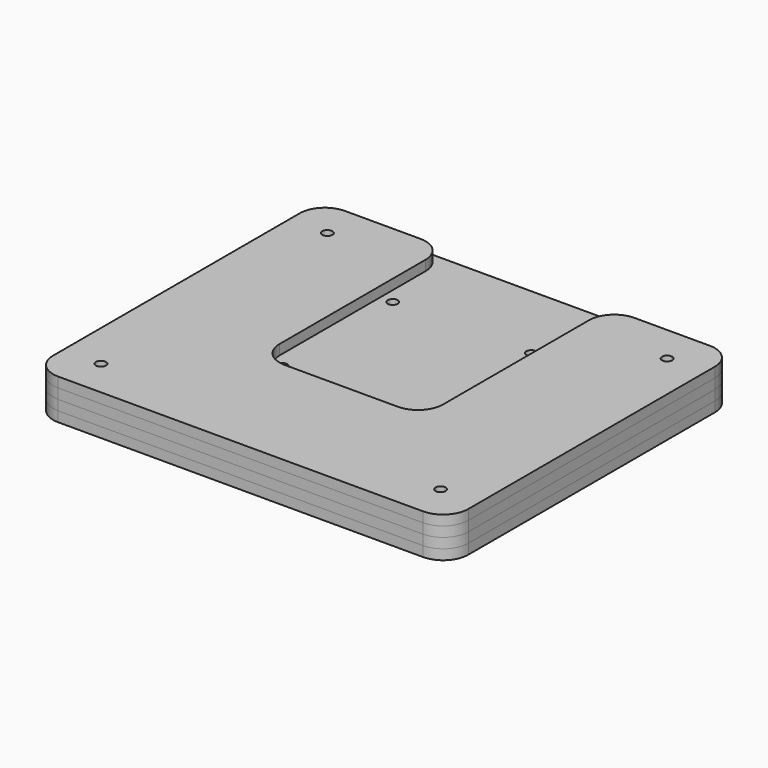
from build123d import *

# Parameters (mm, degrees)
F0_W          = 120
F0_H          = 120
F0_R          = 2
F1_DEPTH      = 4
F2_R          = 10
F3_R          = 4
F4_DEPTH      = 4
F5_W          = 75
F5_H          = 75
F6_DEPTH      = 4
F7_R          = 10
F9_DEPTH      = 4
F10_R         = 4
F10_R_2       = 2
F11_DEPTH     = 4
F12_DEPTH     = 16.001
F13_R         = 2
F14_DEPTH     = 4
F16_DEPTH     = 4
F17_R         = 10
F19_DEPTH     = 4
F20_R         = 10
F22_DEPTH     = 4
F24_DEPTH     = 4
F25_R         = 2
F26_DEPTH     = 16.001
F27_R         = 5
F28_DEPTH     = 8
F30_R         = 2
F31_DEPTH     = 4
F32_TEXT_SIZE = 22.9472929365
F33_DEPTH     = 1
F34_TEXT_SIZE = 22.9472929365
F35_DEPTH     = 1
F36_TEXT_SIZE = 22.9472929365
F37_DEPTH     = 1
F38_TEXT_SIZE = 22.9472929365
F39_DEPTH     = 1
F40_TEXT_SIZE = 22.9472929365
F41_DEPTH     = 1
F42_TEXT_SIZE = 22.9472929365
F43_DEPTH     = 1
F44_TEXT_SIZE = 20.3196105408
F45_DEPTH     = 1
F46_TEXT_SIZE = 20.3196105408
F47_DEPTH     = 1
F48_TEXT_SIZE = 20.3196105408
F49_DEPTH     = 1
F50_TEXT_SIZE = 20.3196105408
F51_DEPTH     = 1


# Not quite as in the source:
# - Text() gives the source's letters only with a copy of the font that has no kerning and outlines rounded to 1/6400 em; it was checked with that copy


with BuildPart() as f1:
    # F0 (on Top) → F1 (new body)
    with BuildSketch(Plane.XY):
        Rectangle(F0_W, F0_H)
        with Locations((-50, -50)):
            Circle(F0_R, mode=Mode.SUBTRACT)
        with Locations((50, -50)):
            Circle(F0_R, mode=Mode.SUBTRACT)
        with Locations((-50, 50)):
            Circle(F0_R, mode=Mode.SUBTRACT)
        with Locations((50, 50)):
            Circle(F0_R, mode=Mode.SUBTRACT)
    extrude(amount=F1_DEPTH)

    # F2
    f2_edges = [f1.edges().sort_by_distance(p)[0] for p in [
        (-60, 60, 2),
        (60, 60, 2),
        (-60, -60, 2),
        (60, -60, 2),
    ]]
    fillet(f2_edges, radius=F2_R)

    # F10 (on face) → F11 (cut, through all)
    with BuildSketch(Plane(origin=(0, 0, 0), x_dir=(1, 0, 0), z_dir=(0, 0, -1))):
        with Locations((27.5, -27.5)):
            Circle(F10_R)
        with Locations((27.5, -27.5)):
            Circle(F10_R_2, mode=Mode.SUBTRACT)
        with Locations((-27.5, -27.5)):
            Circle(F10_R)
        with Locations((-27.5, -27.5)):
            Circle(F10_R_2, mode=Mode.SUBTRACT)
        with Locations((-27.5, 27.5)):
            Circle(F10_R)
        with Locations((-27.5, 27.5)):
            Circle(F10_R_2, mode=Mode.SUBTRACT)
        with Locations((27.5, 27.5)):
            Circle(F10_R)
        with Locations((27.5, 27.5)):
            Circle(F10_R_2, mode=Mode.SUBTRACT)
        with Locations((27.5, -27.5)):
            Circle(F10_R_2)
        with Locations((-27.5, -27.5)):
            Circle(F10_R_2)
        with Locations((-27.5, 27.5)):
            Circle(F10_R_2)
        with Locations((27.5, 27.5)):
            Circle(F10_R_2)
    extrude(amount=-F11_DEPTH, mode=Mode.SUBTRACT)


with BuildPart() as f4:
    # F3 (on face) → F4 (new body)
    with BuildSketch(Plane.XY.offset(4)):
        with BuildLine():
            ThreePointArc((-60, -50), (-57.0710678119, -57.0710678119), (-50, -60))
            Line((-50, -60), (50, -60))
            ThreePointArc((50, -60), (57.0710678119, -57.0710678119), (60, -50))
            Line((60, -50), (60, 50))
            ThreePointArc((60, 50), (57.0710678119, 57.0710678119), (50, 60))
            Line((50, 60), (-50, 60))
            ThreePointArc((-50, 60), (-57.0710678119, 57.0710678119), (-60, 50))
            Line((-60, 50), (-60, -50))
        make_face()
        with Locations((-50, -50)):
            Circle(F3_R, mode=Mode.SUBTRACT)
        with Locations((50, -50)):
            Circle(F3_R, mode=Mode.SUBTRACT)
        with Locations((-50, 50)):
            Circle(F3_R, mode=Mode.SUBTRACT)
        with Locations((50, 50)):
            Circle(F3_R, mode=Mode.SUBTRACT)
    extrude(amount=F4_DEPTH)


with BuildPart() as f6:
    # F5 (on face) → F6 (new body)
    with BuildSketch(Plane.XY.offset(8)):
        Rectangle(F5_W, F5_H)
    extrude(amount=F6_DEPTH)

    # F7
    f7_edges = [f6.edges().sort_by_distance(p)[0] for p in [
        (-37.5, 37.5, 10),
        (37.5, 37.5, 10),
        (37.5, -37.5, 10),
        (-37.5, -37.5, 10),
    ]]
    fillet(f7_edges, radius=F7_R)


with BuildPart() as f9:
    # F8 (on face) → F9 (new body)
    with BuildSketch(Plane.XY.offset(12)):
        with BuildLine():
            ThreePointArc((-60, -50), (-57.0710678119, -57.0710678119), (-50, -60))
            Line((-50, -60), (50, -60))
            ThreePointArc((50, -60), (57.0710678119, -57.0710678119), (60, -50))
            Line((60, -50), (60, 50))
            ThreePointArc((60, 50), (57.0710678119, 57.0710678119), (50, 60))
            Line((50, 60), (-50, 60))
            ThreePointArc((-50, 60), (-57.0710678119, 57.0710678119), (-60, 50))
            Line((-60, 50), (-60, -50))
        make_face()
    extrude(amount=F9_DEPTH)


with BuildPart() as f12_tool:
    # F10 (on face) → F12 (new body, through all)
    with BuildSketch(Plane(origin=(0, 0, 0), x_dir=(1, 0, 0), z_dir=(0, 0, -1))):
        with Locations((27.5, -27.5)):
            Circle(F10_R_2)
        with Locations((-27.5, -27.5)):
            Circle(F10_R_2)
        with Locations((-27.5, 27.5)):
            Circle(F10_R_2)
        with Locations((27.5, 27.5)):
            Circle(F10_R_2)
    extrude(amount=-F12_DEPTH)


with BuildPart() as f4_1:
    add(f4.part)

    # F12: cut by f12_tool
    add(f12_tool.part, mode=Mode.SUBTRACT)

    # F36 (on face) → F37 (cut)
    with BuildSketch(Plane(origin=(0, 0, 4), x_dir=(1, 0, 0), z_dir=(0, 0, -1))):
        with Locations((-15, -8.2610254572)):
            Text('3-1', F36_TEXT_SIZE, font='Open Sans', text_align=(TextAlign.LEFT, TextAlign.BOTTOM))
    extrude(amount=-F37_DEPTH, mode=Mode.SUBTRACT)


with BuildPart() as f6_1:
    add(f6.part)

    # F12: cut by f12_tool
    add(f12_tool.part, mode=Mode.SUBTRACT)

    # F38 (on face) → F39 (cut)
    with BuildSketch(Plane(origin=(0, 0, 8), x_dir=(1, 0, 0), z_dir=(0, 0, -1))):
        with Locations((-15, -8.2610254572)):
            Text('4-1', F38_TEXT_SIZE, font='Open Sans', text_align=(TextAlign.LEFT, TextAlign.BOTTOM))
    extrude(amount=-F39_DEPTH, mode=Mode.SUBTRACT)


with BuildPart() as f9_1:
    add(f9.part)

    # F12: cut by f12_tool
    add(f12_tool.part, mode=Mode.SUBTRACT)


with BuildPart() as f14:
    # F13 (on face) → F14 (new body)
    with BuildSketch(Plane.XY.offset(16)):
        with BuildLine():
            ThreePointArc((-50, 60), (-57.0710678119, 57.0710678119), (-60, 50))
            Line((-60, 50), (-60, -50))
            ThreePointArc((-60, -50), (-57.0710678119, -57.0710678119), (-50, -60))
            Line((-50, -60), (50, -60))
            ThreePointArc((50, -60), (57.0710678119, -57.0710678119), (60, -50))
            Line((60, -50), (60, 50))
            ThreePointArc((60, 50), (57.0710678119, 57.0710678119), (50, 60))
            Line((50, 60), (-50, 60))
        make_face()
        with Locations((-27.5, -27.5)):
            Circle(F13_R, mode=Mode.SUBTRACT)
        with Locations((27.5, -27.5)):
            Circle(F13_R, mode=Mode.SUBTRACT)
        with Locations((-27.5, 27.5)):
            Circle(F13_R, mode=Mode.SUBTRACT)
        with Locations((27.5, 27.5)):
            Circle(F13_R, mode=Mode.SUBTRACT)
    extrude(amount=F14_DEPTH)


with BuildPart() as f16:
    # F15 (on face) → F16 (new body)
    with BuildSketch(Plane.XY.offset(20)):
        Polygon((32.5, -32.5), (0, -32.5), (-32.5, -32.5), (-32.5, 60), (-82.5, 60), (-82.5, -82.5), (0, -82.5), (82.5, -82.5), (82.5, 60), (32.5, 60), align=None)
    extrude(amount=F16_DEPTH)

    # F17
    f17_edges = [f16.edges().sort_by_distance(p)[0] for p in [
        (-32.5, 60, 22),
        (82.5, 60, 22),
        (82.5, -82.5, 22),
        (-32.5, -32.5, 22),
        (-82.5, 60, 22),
        (32.5, 60, 22),
        (32.5, -32.5, 22),
        (-82.5, -82.5, 22),
    ]]
    fillet(f17_edges, radius=F17_R)


with BuildPart() as f19:
    # F18 (on face) → F19 (new body)
    with BuildSketch(Plane(origin=(0, 0, 20), x_dir=(1, 0, 0), z_dir=(0, 0, -1))):
        with BuildLine():
            ThreePointArc((50, 60), (57.0710678119, 57.0710678119), (60, 50))
            Line((60, 50), (60, -50))
            Line((60, -50), (60, -60))
            Line((60, -60), (72.5, -60))
            ThreePointArc((72.5, -60), (79.5710678119, -57.0710678119), (82.5, -50))
            Line((82.5, -50), (82.5, 72.5))
            ThreePointArc((82.5, 72.5), (79.5710678119, 79.5710678119), (72.5, 82.5))
            Line((72.5, 82.5), (-72.5, 82.5))
            ThreePointArc((-72.5, 82.5), (-79.5710678119, 79.5710678119), (-82.5, 72.5))
            Line((-82.5, 72.5), (-82.5, -50))
            ThreePointArc((-82.5, -50), (-79.5710678119, -57.0710678119), (-72.5, -60))
            Line((-72.5, -60), (-60, -60))
            Line((-60, -60), (-60, -50))
            Line((-60, -50), (-60, 50))
            ThreePointArc((-60, 50), (-57.0710678119, 57.0710678119), (-50, 60))
            Line((-50, 60), (50, 60))
        make_face()
    extrude(amount=F19_DEPTH)

    # F20
    f20_edges = [f19.edges().sort_by_distance(p)[0] for p in [
        (-60, 60, 18),
        (60, 60, 18),
    ]]
    fillet(f20_edges, radius=F20_R)


with BuildPart() as f22:
    # F21 (on face) → F22 (new body)
    with BuildSketch(Plane(origin=(0, 0, 16), x_dir=(1, 0, 0), z_dir=(0, 0, -1))):
        with BuildLine():
            ThreePointArc((50, 60), (57.0710678119, 57.0710678119), (60, 50))
            Line((60, 50), (60, -50))
            ThreePointArc((60, -50), (62.9289321881, -57.0710678119), (70, -60))
            Line((70, -60), (72.5, -60))
            ThreePointArc((72.5, -60), (79.5710678119, -57.0710678119), (82.5, -50))
            Line((82.5, -50), (82.5, 72.5))
            ThreePointArc((82.5, 72.5), (79.5710678119, 79.5710678119), (72.5, 82.5))
            Line((72.5, 82.5), (-72.5, 82.5))
            ThreePointArc((-72.5, 82.5), (-79.5710678119, 79.5710678119), (-82.5, 72.5))
            Line((-82.5, 72.5), (-82.5, -50))
            ThreePointArc((-82.5, -50), (-79.5710678119, -57.0710678119), (-72.5, -60))
            Line((-72.5, -60), (-70, -60))
            ThreePointArc((-70, -60), (-62.9289321881, -57.0710678119), (-60, -50))
            Line((-60, -50), (-60, 50))
            ThreePointArc((-60, 50), (-57.0710678119, 57.0710678119), (-50, 60))
            Line((-50, 60), (50, 60))
        make_face()
    extrude(amount=F22_DEPTH)


with BuildPart() as f24:
    # F23 (on face) → F24 (new body)
    with BuildSketch(Plane(origin=(0, 0, 12), x_dir=(1, 0, 0), z_dir=(0, 0, -1))):
        with BuildLine():
            Line((47.5, -60), (70, -60))
            Line((70, -60), (72.5, -60))
            ThreePointArc((72.5, -60), (79.5710678119, -57.0710678119), (82.5, -50))
            Line((82.5, -50), (82.5, 72.5))
            ThreePointArc((82.5, 72.5), (79.5710678119, 79.5710678119), (72.5, 82.5))
            Line((72.5, 82.5), (-72.5, 82.5))
            ThreePointArc((-72.5, 82.5), (-79.5710678119, 79.5710678119), (-82.5, 72.5))
            Line((-82.5, 72.5), (-82.5, -50))
            ThreePointArc((-82.5, -50), (-79.5710678119, -57.0710678119), (-72.5, -60))
            Line((-72.5, -60), (-70, -60))
            Line((-70, -60), (-47.5, -60))
            ThreePointArc((-47.5, -60), (-40.4289321881, -57.0710678119), (-37.5, -50))
            Line((-37.5, -50), (-37.5, -27.5))
            Line((-37.5, -27.5), (-37.5, 27.5))
            ThreePointArc((-37.5, 27.5), (-34.5710678119, 34.5710678119), (-27.5, 37.5))
            Line((-27.5, 37.5), (27.5, 37.5))
            ThreePointArc((27.5, 37.5), (34.5710678119, 34.5710678119), (37.5, 27.5))
            Line((37.5, 27.5), (37.5, -27.5))
            Line((37.5, -27.5), (37.5, -50))
            ThreePointArc((37.5, -50), (40.4289321881, -57.0710678119), (47.5, -60))
        make_face()
    extrude(amount=F24_DEPTH)


with BuildPart() as f26_tool:
    # F25 (on face) → F26 (new body, through all)
    with BuildSketch(Plane(origin=(0, 0, 8), x_dir=(1, 0, 0), z_dir=(0, 0, -1))):
        with Locations((-67.5, 67.5)):
            Circle(F25_R)
        with Locations((67.5, 67.5)):
            Circle(F25_R)
        with Locations((67.5, -45)):
            Circle(F25_R)
        with Locations((-67.5, -45)):
            Circle(F25_R)
    extrude(amount=-F26_DEPTH)


with BuildPart() as f16_1:
    add(f16.part)

    # F26: cut by f26_tool
    add(f26_tool.part, mode=Mode.SUBTRACT)

    # F50 (on face) → F51 (cut)
    with BuildSketch(Plane(origin=(0, 0, 20), x_dir=(1, 0, 0), z_dir=(0, 0, -1))):
        with Locations((-15, 50.1849402053)):
            Text('4-2', F50_TEXT_SIZE, font='Open Sans', text_align=(TextAlign.LEFT, TextAlign.BOTTOM))
    extrude(amount=-F51_DEPTH, mode=Mode.SUBTRACT)


with BuildPart() as f19_1:
    add(f19.part)

    # F26: cut by f26_tool
    add(f26_tool.part, mode=Mode.SUBTRACT)

    # F48 (on face) → F49 (cut)
    with BuildSketch(Plane(origin=(0, 0, 16), x_dir=(1, 0, 0), z_dir=(0, 0, -1))):
        with Locations((-15, 63.9349402053)):
            Text('3-2', F48_TEXT_SIZE, font='Open Sans', text_align=(TextAlign.LEFT, TextAlign.BOTTOM))
    extrude(amount=-F49_DEPTH, mode=Mode.SUBTRACT)


with BuildPart() as f22_1:
    add(f22.part)

    # F26: cut by f26_tool
    add(f26_tool.part, mode=Mode.SUBTRACT)

    # F46 (on face) → F47 (cut)
    with BuildSketch(Plane(origin=(0, 0, 12), x_dir=(1, 0, 0), z_dir=(0, 0, -1))):
        with Locations((-15, 63.9349402053)):
            Text('2-2', F46_TEXT_SIZE, font='Open Sans', text_align=(TextAlign.LEFT, TextAlign.BOTTOM))
    extrude(amount=-F47_DEPTH, mode=Mode.SUBTRACT)


with BuildPart() as f24_1:
    add(f24.part)

    # F26: cut by f26_tool
    add(f26_tool.part, mode=Mode.SUBTRACT)

    # F44 (on face) → F45 (cut)
    with BuildSketch(Plane(origin=(0, 0, 8), x_dir=(1, 0, 0), z_dir=(0, 0, -1))):
        with Locations((-15, 52.6849402053)):
            Text('1-2', F44_TEXT_SIZE, font='Open Sans', text_align=(TextAlign.LEFT, TextAlign.BOTTOM))
    extrude(amount=-F45_DEPTH, mode=Mode.SUBTRACT)


with BuildPart() as f28_tool:
    # F27 (on face) → F28 (new body, through all)
    with BuildSketch(Plane.XY.offset(20)):
        with Locations((-50, 50)):
            Circle(F27_R)
        with Locations((50, 50)):
            Circle(F27_R)
        with Locations((-50, -50)):
            Circle(F27_R)
        with Locations((50, -50)):
            Circle(F27_R)
    extrude(amount=-F28_DEPTH)


with BuildPart() as f9_2:
    add(f9_1.part)

    # F28: cut by f28_tool
    add(f28_tool.part, mode=Mode.SUBTRACT)

    # F40 (on face) → F41 (cut)
    with BuildSketch(Plane(origin=(0, 0, 12), x_dir=(1, 0, 0), z_dir=(0, 0, -1))):
        with Locations((-15, -8.2610254572)):
            Text('5-1', F40_TEXT_SIZE, font='Open Sans', text_align=(TextAlign.LEFT, TextAlign.BOTTOM))
    extrude(amount=-F41_DEPTH, mode=Mode.SUBTRACT)


with BuildPart() as f14_1:
    add(f14.part)

    # F28: cut by f28_tool
    add(f28_tool.part, mode=Mode.SUBTRACT)

    # F42 (on face) → F43 (join)
    with BuildSketch(Plane(origin=(0, 0, 16), x_dir=(1, 0, 0), z_dir=(0, 0, -1))):
        with Locations((-15, -8.2610254572)):
            Text('6-1', F42_TEXT_SIZE, font='Open Sans', text_align=(TextAlign.LEFT, TextAlign.BOTTOM))
    extrude(amount=F43_DEPTH)


with BuildPart() as f1_1:
    # F29: moved
    add(f1.part.moved(Location((0, 0, -4))))

    # F32 (on face) → F33 (cut)
    with BuildSketch(Plane(origin=(0, 0, -4), x_dir=(1, 0, 0), z_dir=(0, 0, -1))):
        with Locations((-15, -8.2610254572)):
            Text('1-1', F32_TEXT_SIZE, font='Open Sans', text_align=(TextAlign.LEFT, TextAlign.BOTTOM))
    extrude(amount=-F33_DEPTH, mode=Mode.SUBTRACT)


with BuildPart() as f31:
    # F30 (on face) → F31 (new body)
    with BuildSketch(Plane(origin=(0, 0, 4), x_dir=(1, 0, 0), z_dir=(0, 0, -1))):
        with BuildLine():
            ThreePointArc((60, 50), (57.0710678119, 57.0710678119), (50, 60))
            Line((50, 60), (-50, 60))
            ThreePointArc((-50, 60), (-57.0710678119, 57.0710678119), (-60, 50))
            Line((-60, 50), (-60, -50))
            ThreePointArc((-60, -50), (-57.0710678119, -57.0710678119), (-50, -60))
            Line((-50, -60), (50, -60))
            ThreePointArc((50, -60), (57.0710678119, -57.0710678119), (60, -50))
            Line((60, -50), (60, 50))
        make_face()
        with Locations((-50, -50)):
            Circle(F30_R, mode=Mode.SUBTRACT)
        with Locations((-27.5, -27.5)):
            Circle(F30_R, mode=Mode.SUBTRACT)
        with Locations((50, -50)):
            Circle(F30_R, mode=Mode.SUBTRACT)
        with Locations((27.5, -27.5)):
            Circle(F30_R, mode=Mode.SUBTRACT)
        with Locations((-27.5, 27.5)):
            Circle(F30_R, mode=Mode.SUBTRACT)
        with Locations((-50, 50)):
            Circle(F30_R, mode=Mode.SUBTRACT)
        with Locations((27.5, 27.5)):
            Circle(F30_R, mode=Mode.SUBTRACT)
        with Locations((50, 50)):
            Circle(F30_R, mode=Mode.SUBTRACT)
    extrude(amount=F31_DEPTH)

    # F34 (on face) → F35 (cut)
    with BuildSketch(Plane(origin=(0, 0, 0), x_dir=(1, 0, 0), z_dir=(0, 0, -1))):
        with Locations((-15, -8.2610254572)):
            Text('2-1', F34_TEXT_SIZE, font='Open Sans', text_align=(TextAlign.LEFT, TextAlign.BOTTOM))
    extrude(amount=-F35_DEPTH, mode=Mode.SUBTRACT)


solid = Compound([f4_1.part, f6_1.part, f16_1.part, f19_1.part, f22_1.part, f24_1.part, f9_2.part, f14_1.part, f1_1.part, f31.part])
